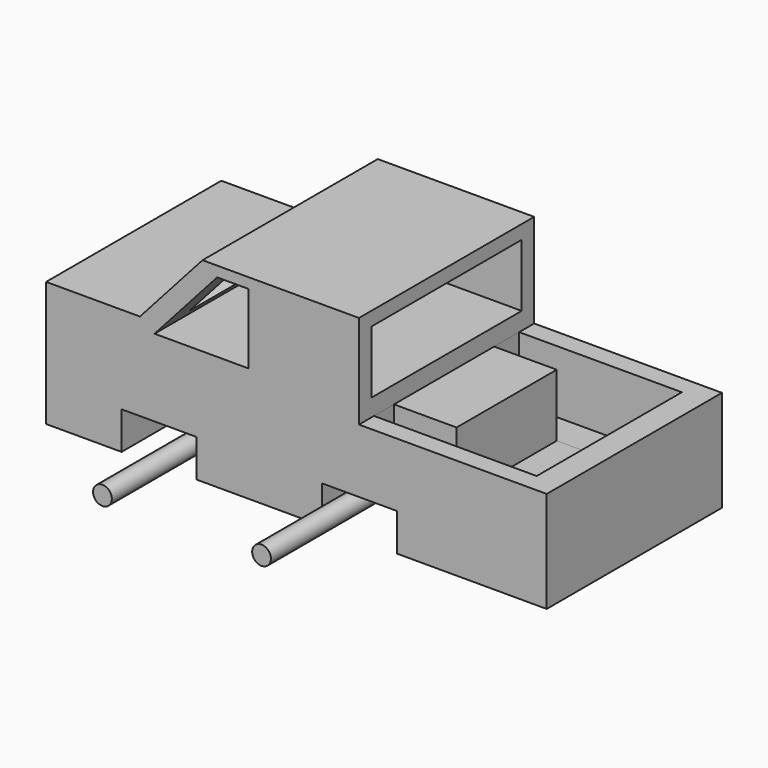
from build123d import *

# Parameters (mm, degrees)
F0_W          = 30.48
F0_H          = 15.24
F1_DEPTH      = 88.9
F2_W          = 30.48
F2_H          = 15.24
F3_DEPTH      = 38.1
F4_W          = 30.48
F4_H          = 15.24
F5_DEPTH      = 38.1
F6_R          = 3.81
F7_DEPTH      = 127
F7_DEPTH_BACK = 38.1
F9_DEPTH      = 88.9
F10_W         = 66.04
F10_H         = 73.66
F11_DEPTH     = 25.4
F12_W         = 63.5
F12_H         = 25.4
F13_DEPTH     = 12.7
F15_W         = 76.2
F15_H         = 25.4
F16_DEPTH     = 50.8
F18_DEPTH     = 7.62
F19_W         = 26.801726786
F19_H         = 6.35
F14_W         = 25.4
F14_H         = 6.35
F20_DEPTH     = 12.7
F21_DEPTH     = 12.7
F22_W         = 50.8
F22_H         = 25.4
F23_DEPTH     = 38.1
F24_DEPTH     = 12.7


# Not quite as in the source:
# - a feature names something its author has since deleted; it is built from what else it names


with BuildPart() as f1:
    # F0 (on Front) → F1 (new body)
    with BuildSketch(Plane.XZ):
        Polygon((0, 50.8), (0, 0), (29.5417681336, 0), (29.5417681336, 15.24), (60.0217681336, 15.24), (60.0217681336, 0), (121.1203709245, 0), (121.1203709245, 15.24), (151.6003709245, 15.24), (151.6003709245, 0), (203.2, 0), (203.2, 41.0980633142), (127, 41.0980633142), (127, 79.1980633142), (63.5, 79.1980633142), (38.1, 50.8), align=None)
        with Locations((44.7817681336, 7.62)):
            Rectangle(F0_W, F0_H)
        with Locations((136.3603709245, 7.62)):
            Rectangle(F0_W, F0_H)
    extrude(amount=F1_DEPTH)

    # F2 (on face) → F3 (cut)
    with BuildSketch(Plane.XZ.offset(88.9)):
        with Locations((45.8910012597, 7.62)):
            Rectangle(F2_W, F2_H)
        with Locations((127.1710012597, 7.62)):
            Rectangle(F2_W, F2_H)
    extrude(amount=-F3_DEPTH, mode=Mode.SUBTRACT)

    # F4 (on face) → F5 (cut)
    with BuildSketch(Plane(origin=(0, 0, 0), x_dir=(-1, 0, 0), z_dir=(0, 1, 0))):
        with Locations((-126.0602, 7.62)):
            Rectangle(F4_W, F4_H)
        with Locations((-44.7802, 7.62)):
            Rectangle(F4_W, F4_H)
    extrude(amount=-F5_DEPTH, mode=Mode.SUBTRACT)

    # F6 (on Front) → F7 (join, two sides)
    with BuildSketch(Plane.XZ) as f7_sk:
        with Locations((53.3541933731, 7.3445781872)):
            Circle(F6_R)
        with Locations((117.9336786941, 6.9635785541)):
            Circle(F6_R)
    extrude(amount=F7_DEPTH)
    extrude(f7_sk.sketch, amount=-F7_DEPTH_BACK)

    # F8 (on Front) → F9 (cut)
    with BuildSketch(Plane.XZ):
        Polygon((69.4312418273, 74.989986462), (44.0312418273, 46.5919231478), (82.1312418273, 46.5919231478), (82.1312418273, 74.989986462), align=None)
    extrude(amount=F9_DEPTH, mode=Mode.SUBTRACT)

    # F10 (on face) → F11 (cut)
    with BuildSketch(Plane.XY.offset(41.0980633142)):
        with Locations((160.02, -44.45)):
            Rectangle(F10_W, F10_H)
    extrude(amount=-F11_DEPTH, mode=Mode.SUBTRACT)

    # F12 (on face) → F13 (cut)
    with BuildSketch(Plane(origin=(-4.0760562793, 0, 3.6457355683), x_dir=(0, -1, 0), z_dir=(-0.7453559925, 0, 0.6666666667))):
        with Locations((43.8565216027, 81.8850251743)):
            Rectangle(F12_W, F12_H)
    extrude(amount=-F13_DEPTH, mode=Mode.SUBTRACT)

    # F15 (on face) → F16 (cut)
    with BuildSketch(Plane.YZ.offset(127)):
        with Locations((-44.45, 60.8695521951)):
            Rectangle(F15_W, F15_H)
    extrude(amount=-F16_DEPTH, mode=Mode.SUBTRACT)

    # F17 (on face) → F18 (join)
    with BuildSketch(Plane(origin=(0, 0, 0), x_dir=(0, -1, 0), z_dir=(-1, 0, 0))):
        Polygon((56.9462627172, 26.2763872743), (56.9462627172, 31.5944552422), (37.3661071062, 31.5944552422), (37.3661071062, 26.0346587747), (24.7961338609, 26.0346587747), (27.4551659822, 18.7827479094), (37.6078411937, 18.7827479094), (37.6078411937, 13.9481425285), (56.7045323551, 13.9481425285), (56.7045323551, 18.7827479094), (68.0658593774, 18.7827479094), (63.7147128582, 26.2763872743), align=None)
    extrude(amount=-F18_DEPTH)

    # F19 (on face) + F14 (on face) → F20 (join)
    with BuildSketch(Plane(origin=(0, 0, 0), x_dir=(0, -1, 0), z_dir=(-1, 0, 0))):
        with Locations((70.2801537674, 38.6348730328)):
            Rectangle(F19_W, F19_H)
    with BuildSketch(Plane(origin=(0, 0, 0), x_dir=(0, -1, 0), z_dir=(-1, 0, 0))):
        with Locations((18.7792903744, 38.6348730328)):
            Rectangle(F14_W, F14_H)
    extrude(amount=F20_DEPTH)

    # F21 (cut): faces of the model
    f21_faces = [f1.faces().sort_by_distance(p)[0] for p in [
        (-12.7, -18.7792903744, 38.6348730328),
        (-12.7, -70.2801537674, 38.6348730328),
    ]]
    extrude(f21_faces, amount=-F21_DEPTH, mode=Mode.SUBTRACT)

    # F22 (on face) → F23 (join)
    with BuildSketch(Plane.YZ.offset(127)):
        with Locations((-45.72, 28.3980633142)):
            Rectangle(F22_W, F22_H)
    extrude(amount=F23_DEPTH)

    # F24 (cut): a face of the model
    f24_faces = [f1.faces().sort_by_distance(p)[0] for p in [
        (165.1, -45.72, 28.3980633142),
    ]]
    extrude(f24_faces, amount=-F24_DEPTH, mode=Mode.SUBTRACT)


solid = f1.part
